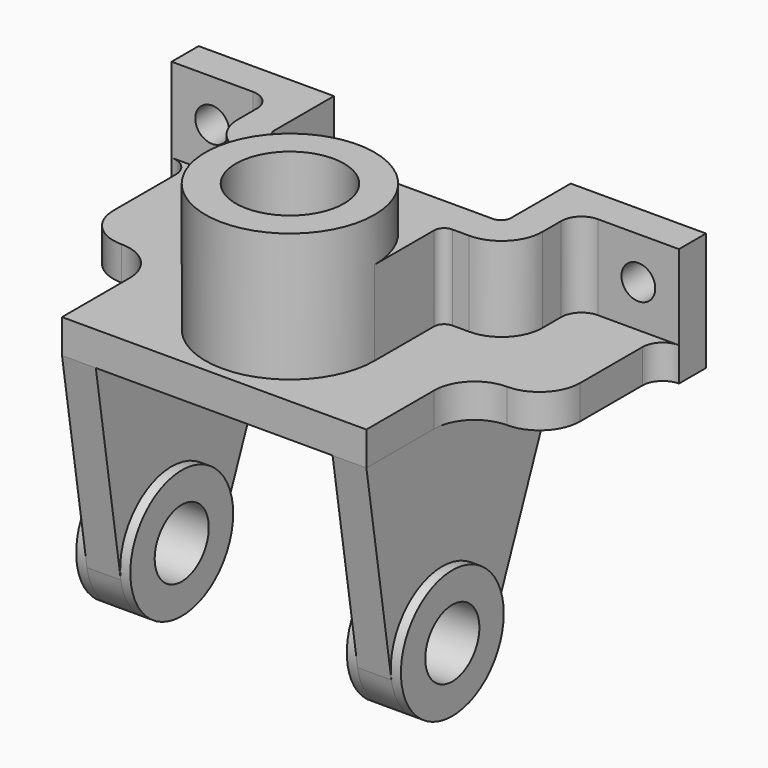
from build123d import *

# Parameters (mm, degrees)
F0_R          = 25
F0_R_2        = 16
F1_DEPTH      = 38
F3_DEPTH      = 25
F3_DEPTH_BACK = 10
F4_R          = 6
F5_R          = 3
F6_R          = 12
F8_DEPTH      = 10
F9_R          = 11.99999
F11_DEPTH     = 10
F12_R         = 19
F13_DEPTH     = 3
F17_D         = 20
F17_DEPTH     = 25
F17_TIP       = 6.0086061903
F20_D         = 10
F20_DEPTH     = 25
F20_TIP       = 3.0043030951


# Not quite as in the source:
# - a fillet or chamfer is up to 0.001 mm smaller than in the source, because OpenCascade refuses the exact size


with BuildPart() as f1:
    # F0 (on Top) → F1 (new body)
    with BuildSketch(Plane.XY):
        Circle(F0_R)
        Circle(F0_R_2, mode=Mode.SUBTRACT)
    extrude(amount=F1_DEPTH)

    # F2 (on Top) → F3 (join, two sides)
    with BuildSketch(Plane.XY) as f3_sk:
        with BuildLine():
            Line((-35, 60), (-75, 60))
            Line((-75, 60), (-75, 50))
            Line((-75, 50), (-45, 50))
            Line((-45, 50), (-45, 25))
            Line((-45, 25), (-25, 25))
            Line((-25, 25), (-25, 0))
            ThreePointArc((-25, 0), (0, 25), (25, 0))
            Line((25, 0), (25, 25))
            Line((25, 25), (45, 25))
            Line((45, 25), (45, 50))
            Line((45, 50), (75, 50))
            Line((75, 50), (75, 60))
            Line((75, 60), (35, 60))
            Line((35, 60), (35, 35))
            Line((35, 35), (0, 35))
            Line((0, 35), (-35, 35))
            Line((-35, 35), (-35, 60))
        make_face()
    extrude(amount=F3_DEPTH)
    extrude(f3_sk.sketch, amount=-F3_DEPTH_BACK)

    # F4
    f4_edges = [f1.edges().sort_by_distance(p)[0] for p in [
        (45, 50, 7.5),
        (-45, 50, 7.5),
    ]]
    fillet(f4_edges, radius=F4_R)

    # F5
    f5_edges = [f1.edges().sort_by_distance(p)[0] for p in [
        (25, 25, 7.5),
        (-25, 25, 7.5),
        (-35, 35, 7.5),
        (35, 35, 7.5),
    ]]
    fillet(f5_edges, radius=F5_R)

    # F6
    f6_edges = [f1.edges().sort_by_distance(p)[0] for p in [
        (-45, 25, 7.5),
        (45, 25, 7.5),
    ]]
    fillet(f6_edges, radius=F6_R)

    # F20
    with Locations(Plane.XZ.offset(-50)):
        with Locations((-63, 12.5), (63, 12.5)):
            Hole(F20_D / 2, depth=F20_DEPTH)
            with Locations((0, 0, -(F20_DEPTH + F20_TIP / 2))):  # 118° drill point
                Cone(0, F20_D / 2, F20_TIP, mode=Mode.SUBTRACT)


with BuildPart() as f8:
    # F7 (on Top) → F8 (new body)
    with BuildSketch(Plane.XY):
        with BuildLine():
            Line((-45, -28), (0, -28))
            Line((0, -28), (45, -28))
            Line((45, -28), (45, 9))
            Line((45, 9), (69, 9))
            Line((69, 9), (69, 44))
            ThreePointArc((69, 44), (70.7573593129, 48.2426406871), (75, 50))
            Line((75, 50), (51, 50))
            ThreePointArc((51, 50), (46.7573593129, 48.2426406871), (45, 44))
            Line((45, 44), (45, 37))
            ThreePointArc((45, 37), (41.4852813742, 28.5147186258), (33, 25))
            Line((33, 25), (28, 25))
            ThreePointArc((28, 25), (25.8786796564, 24.1213203436), (25, 22))
            Line((25, 22), (25, 0))
            ThreePointArc((25, 0), (0, -25), (-25, 0))
            Line((-25, 0), (-25, 22))
            ThreePointArc((-25, 22), (-25.8786796564, 24.1213203436), (-28, 25))
            Line((-28, 25), (-33, 25))
            ThreePointArc((-33, 25), (-41.4852813742, 28.5147186258), (-45, 37))
            Line((-45, 37), (-45, 44))
            ThreePointArc((-45, 44), (-46.7573593129, 48.2426406871), (-51, 50))
            Line((-51, 50), (-75, 50))
            ThreePointArc((-75, 50), (-70.7573593129, 48.2426406871), (-69, 44))
            Line((-69, 44), (-69, 9))
            Line((-69, 9), (-45, 9))
            Line((-45, 9), (-45, -28))
        make_face()
    extrude(amount=-F8_DEPTH)

    # F9 (radius 12 in the source; OpenCascade refuses exactly that, so slightly less here)
    f9_edges = [f8.edges().sort_by_distance(p)[0] for p in [
        (-69, 9, -5),
        (-45, 9, -5),
        (45, 9, -5),
        (69, 9, -5),
    ]]
    fillet(f9_edges, radius=F9_R)


with BuildPart() as f11:
    # F10 (on face) → F11 (new body)
    with BuildSketch(Plane.YZ.offset(45)):
        with BuildLine():
            Line((-28, -10), (-18.7712820587, -68.9392124579))
            ThreePointArc((-18.7712820587, -68.9392124579), (-2.1708355833, -84.8755787427), (17.6139596592, -73.1237928888))
            Line((17.6139596592, -73.1237928888), (36.8237372905, -25.6265883042))
            ThreePointArc((36.8237372905, -25.6265883042), (46.0238648475, -14.2715739575), (60, -10))
            Line((60, -10), (50, -10))
            Line((50, -10), (44, -10))
            Line((44, -10), (21, -10))
            Line((21, -10), (9, -10))
            Line((9, -10), (-3, -10))
            Line((-3, -10), (-28, -10))
        make_face()
    extrude(amount=-F11_DEPTH)

    # F12 (on face) → F13 (join)
    with BuildSketch(Plane.YZ.offset(45)):
        with Locations((0, -66)):
            Circle(F12_R)
    extrude(amount=F13_DEPTH)

    # F15: F11 across plane


with BuildPart() as f11_1:
    add(f11.part)
    add(f11.part.mirror(Plane(origin=(40, 0, -66), x_dir=(0, 1, 0), z_dir=(1, 0, 0))))

    # F17
    with Locations(Plane.YZ.offset(48)):
        with Locations((0, -66)):
            Hole(F17_D / 2, depth=F17_DEPTH)
            with Locations((0, 0, -(F17_DEPTH + F17_TIP / 2))):  # 118° drill point
                Cone(0, F17_D / 2, F17_TIP, mode=Mode.SUBTRACT)


with BuildPart() as f18_1:
    # F18: instance of F11
    add(f11_1.part.mirror(Plane.YZ))


solid = Compound([f1.part, f8.part, f11_1.part, f18_1.part])
